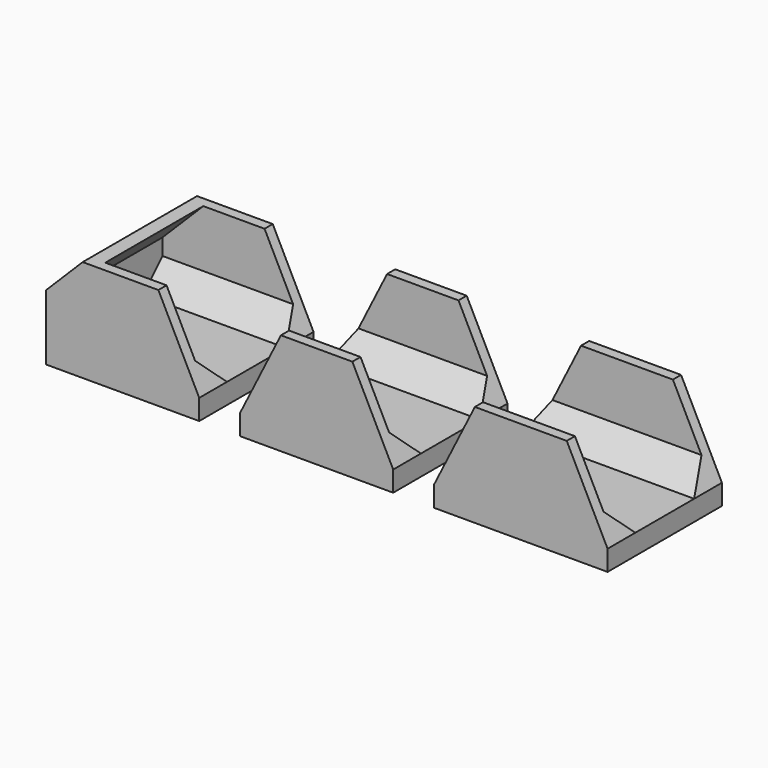
from build123d import *

# Parameters (mm, degrees)
F0_W      = 9.525
F0_H      = 12.7
F1_DEPTH  = 11.1125
F0_W_2    = 11.1125
F0_W_3    = 14.2875
F2_DEPTH  = 9.525
F3_SIZE   = 3.81
F3_2_SIZE = 3.81
F3_3_SIZE = 3.81


# Not quite as in the source:
# - a feature names something its author has since deleted; it is built from what else it names


with BuildPart() as f1:
    # F0 (on Front) → F1 (new body, symmetric)
    with BuildSketch(Plane.XZ):
        Polygon((-46.83125, 0), (-40.48125, 0), (-40.48125, 12.7), (-46.83125, 6.35), align=None)
        Polygon((-30.95625, 0), (-24.60625, 0), (-30.95625, 12.7), align=None)
        Polygon((-48.41875, -3.175), (-46.83125, -3.175), (-46.83125, 0), (-46.83125, 6.35), (-40.48125, 12.7), (-42.7263140303, 12.7), (-48.41875, 7.0075640303), (-48.41875, 6.35), align=None)
        Polygon((-24.60625, -3.175), (-24.60625, 0), (-30.95625, 0), (-40.48125, 0), (-46.83125, 0), (-46.83125, -3.175), align=None)
        with Locations((-35.71875, 6.35)):
            Rectangle(F0_W, F0_H)
    extrude(amount=F1_DEPTH, both=True)


with BuildPart() as f1b:
    # F0 (on Front) → F1, piece 2 (new body, symmetric)
    with BuildSketch(Plane.XZ):
        Polygon((-18.25625, 0), (-11.90625, 0), (-11.90625, 12.7), align=None)
        Polygon((-0.79375, 0), (5.55625, 0), (-0.79375, 12.7), align=None)
        Polygon((5.55625, -3.175), (5.55625, 0), (-0.79375, 0), (-11.90625, 0), (-18.25625, 0), (-18.25625, -3.175), align=None)
        with Locations((-6.35, 6.35)):
            Rectangle(F0_W_2, F0_H)
    extrude(amount=F1_DEPTH, both=True)


with BuildPart() as f1c:
    # F0 (on Front) → F1, piece 3 (new body, symmetric)
    with BuildSketch(Plane.XZ):
        Polygon((18.25625, 12.7), (11.90625, 0), (18.25625, 0), align=None)
        Polygon((32.54375, 0), (38.89375, 0), (32.54375, 12.7), align=None)
        Polygon((11.90625, 0), (11.90625, -3.175), (38.89375, -3.175), (38.89375, 0), (32.54375, 0), (18.25625, 0), align=None)
        with Locations((25.4, 6.35)):
            Rectangle(F0_W_3, F0_H)
    extrude(amount=F1_DEPTH, both=True)


with BuildPart() as f2_tool:
    # F0 (on Front) → F2 (new body, symmetric)
    with BuildSketch(Plane.XZ):
        Polygon((-46.83125, 0), (-40.48125, 0), (-40.48125, 12.7), (-46.83125, 6.35), align=None)
        with Locations((-35.71875, 6.35)):
            Rectangle(F0_W, F0_H)
        Polygon((-30.95625, 0), (-24.60625, 0), (-30.95625, 12.7), align=None)
        with Locations((-6.35, 6.35)):
            Rectangle(F0_W_2, F0_H)
        Polygon((-18.25625, 0), (-11.90625, 0), (-11.90625, 12.7), align=None)
        Polygon((-0.79375, 0), (5.55625, 0), (-0.79375, 12.7), align=None)
        Polygon((18.25625, 12.7), (11.90625, 0), (18.25625, 0), align=None)
        with Locations((25.4, 6.35)):
            Rectangle(F0_W_3, F0_H)
        Polygon((32.54375, 0), (38.89375, 0), (32.54375, 12.7), align=None)
    extrude(amount=F2_DEPTH, both=True)


with BuildPart() as f1_1:
    add(f1.part)

    # F2: cut by f2_tool
    add(f2_tool.part, mode=Mode.SUBTRACT)

    # F3
    f3_edges = [f1_1.edges().sort_by_distance(p)[0] for p in [
        (-35.71875, -9.525, 0),
        (-35.71875, 9.525, 0),
    ]]
    chamfer(f3_edges, length=F3_SIZE)


with BuildPart() as f1b_1:
    add(f1b.part)

    # F2: cut by f2_tool
    add(f2_tool.part, mode=Mode.SUBTRACT)

    # F3#2
    f3_2_edges = [f1b_1.edges().sort_by_distance(p)[0] for p in [
        (-6.35, 9.525, 0),
        (-6.35, -9.525, 0),
    ]]
    chamfer(f3_2_edges, length=F3_2_SIZE)


with BuildPart() as f1c_1:
    add(f1c.part)

    # F2: cut by f2_tool
    add(f2_tool.part, mode=Mode.SUBTRACT)

    # F3#3
    f3_3_edges = [f1c_1.edges().sort_by_distance(p)[0] for p in [
        (25.4, 9.525, 0),
        (25.4, -9.525, 0),
    ]]
    chamfer(f3_3_edges, length=F3_3_SIZE)


solid = Compound([f1_1.part, f1b_1.part, f1c_1.part])
